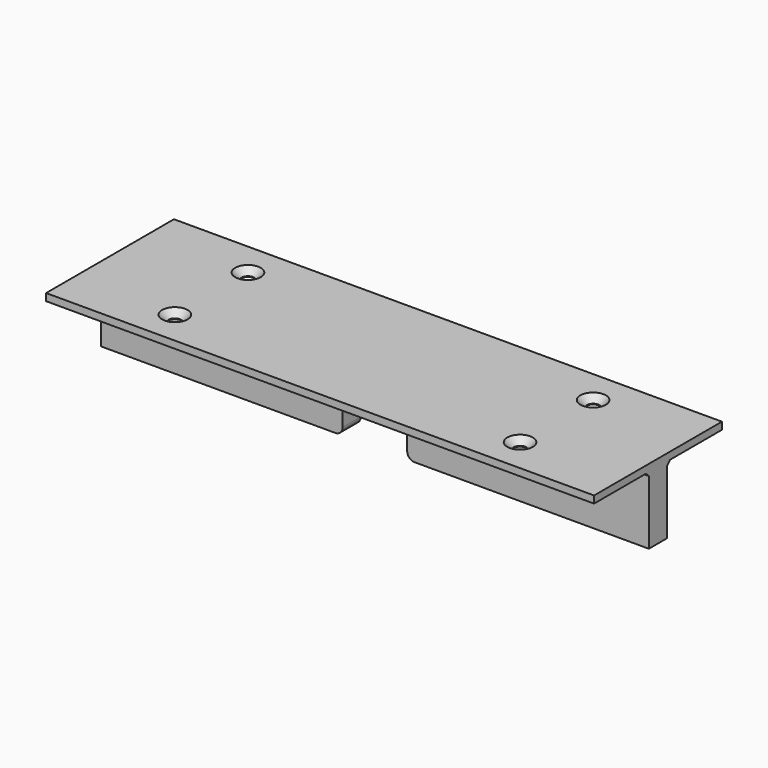
from build123d import *

# Parameters (mm, degrees)
F0_W         = 152.4
F0_H         = 44.45
F1_DEPTH     = 2
F2_W         = 152.4
F2_H         = 6.35
F3_DEPTH     = 18.796
F4_R         = 1.75
F5_DEPTH     = 25
F7_DEPTH     = 25.401
F8_SIZE      = 1.8
F9_T4_DEPTH  = 152.4
F9_S5_R      = 9
F9_T6_DEPTH  = 78
F9_T10_DEPTH = 152.4
F9_S11_R     = 9
F9_T12_DEPTH = 78
F10_R        = 2


# Not quite as in the source:
# - a fillet or chamfer that OpenCascade refuses, or shapes differently, is made with other operations: its cross-section is extruded or revolved along the edge and cut away or added
# - a feature names something its author has since deleted; it is built from what else it names


with BuildPart() as f1:
    # F0 (on Top) → F1 (new body)
    with BuildSketch(Plane.XY):
        Rectangle(F0_W, F0_H)
    extrude(amount=F1_DEPTH)

    # F2 (on face) → F3 (join)
    with BuildSketch(Plane(origin=(0, 0, 0), x_dir=(1, 0, 0), z_dir=(0, 0, -1))):
        Rectangle(F2_W, F2_H)
    extrude(amount=F3_DEPTH)

    # F4 (on face) → F5 (cut)
    with BuildSketch(Plane(origin=(0, 0, 0), x_dir=(1, 0, 0), z_dir=(0, 0, -1))):
        with Locations((48, -12.7)):
            Circle(F4_R)
        with Locations((-48, -12.7)):
            Circle(F4_R)
        with Locations((-48, 12.7)):
            Circle(F4_R)
        with Locations((48, 12.7)):
            Circle(F4_R)
    extrude(amount=-F5_DEPTH, mode=Mode.SUBTRACT)

    # F6 (on face) → F7 (cut, through all)
    with BuildSketch(Plane(origin=(0, 3.175, 0), x_dir=(-1, 0, 0), z_dir=(0, 1, 0))):
        with BuildLine():
            ThreePointArc((-9, -9.398), (0, -18.398), (9, -9.398))
            ThreePointArc((9, -9.398), (0, -0.398), (-9, -9.398))
        make_face()
        with BuildLine():
            Line((9, -18.796), (9, -9.398))
            ThreePointArc((9, -9.398), (0, -18.398), (-9, -9.398))
            Line((-9, -9.398), (-9, -18.796))
            Line((-9, -18.796), (9, -18.796))
        make_face()
    extrude(amount=-F7_DEPTH, mode=Mode.SUBTRACT)

    # F8
    f8_edges = [f1.edges().sort_by_distance(p)[0] for p in [
        (46.25, -12.7, 2),
        (-49.75, -12.7, 2),
        (-49.75, 12.7, 2),
        (46.25, 12.7, 2),
    ]]
    chamfer(f8_edges, length=F8_SIZE)

    # F9: chamfer of 1 on 2 edges, made by hand


with BuildPart() as f9_tool2:
    # F9_s3 → F9_t4 (new body)
    with BuildSketch(Plane.YZ.offset(-76.2)):
        Polygon((3.175, -1), (4.175, 0), (3.175, 0), align=None)
    extrude(amount=F9_T4_DEPTH)

    # F9_s5 → F9_t6 (cut, symmetric)
    with BuildSketch(Plane.XZ.offset(-3.7)):
        with Locations((0, -9.398)):
            Circle(F9_S5_R)
    extrude(amount=F9_T6_DEPTH, both=True, mode=Mode.SUBTRACT)


with BuildPart() as f1_1:
    add(f1.part)

    # F9_t1: union F9_tool2
    add(f9_tool2.part)


with BuildPart() as f9_tool8:
    # F9_s9 → F9_t10 (new body)
    with BuildSketch(Plane.YZ.offset(76.2)):
        Polygon((-4.175, 0), (-3.175, -1), (-3.175, 0), align=None)
    extrude(amount=-F9_T10_DEPTH)

    # F9_s11 → F9_t12 (cut, symmetric)
    with BuildSketch(Plane.XZ.offset(3.7)):
        with Locations((0, -9.398)):
            Circle(F9_S11_R)
    extrude(amount=F9_T12_DEPTH, both=True, mode=Mode.SUBTRACT)


with BuildPart() as f1_2:
    add(f1_1.part)

    # F9_t7: union F9_tool8
    add(f9_tool8.part)

    # F10
    f10_edges = [f1_2.edges().sort_by_distance(p)[0] for p in [
        (9, 0, -18.796),
        (-9, 0, -18.796),
    ]]
    fillet(f10_edges, radius=F10_R)


solid = f1_2.part
